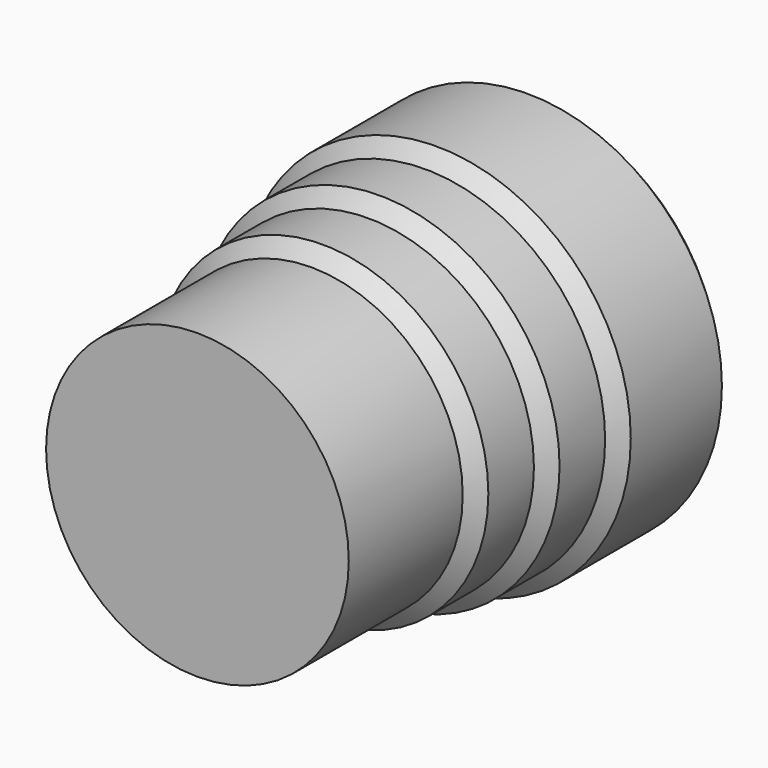
from build123d import *

# Parameters (mm, degrees)
F0_R     = 69.2237369755
F1_DEPTH = 50.8
F2_SIZE  = 5.08
F3_DEPTH = 25.4
F4_SIZE  = 5.08
F5_DEPTH = 25.4
F6_SIZE  = 5.08
F7_DEPTH = 50.8


with BuildPart() as f1:
    # F0 (on Front) → F1 (new body)
    with BuildSketch(Plane.XZ):
        with Locations((-16.0285290331, 36.5865901113)):
            Circle(F0_R)
    extrude(amount=F1_DEPTH)

    # F2
    f2_edges = [f1.edges().sort_by_distance(p)[0] for p in [
        (53.195208, -25.4, 36.58659),
        (-85.252266, 0, 36.58659),
        (-85.252266, -50.8, 36.58659),
    ]]
    chamfer(f2_edges, length=F2_SIZE)

    # F3 (add): a face of the model
    f3_faces = [f1.faces().sort_by_distance(p)[0] for p in [
        (-16.0285290331, -50.8, 36.5865901113),
    ]]
    extrude(f3_faces, amount=F3_DEPTH)

    # F4
    f4_edges = [f1.edges().sort_by_distance(p)[0] for p in [
        (-80.172266, -76.2, 36.58659),
    ]]
    chamfer(f4_edges, length=F4_SIZE)

    # F5 (add): a face of the model
    f5_faces = [f1.faces().sort_by_distance(p)[0] for p in [
        (-16.0285290331, -76.2, 36.5865901113),
    ]]
    extrude(f5_faces, amount=F5_DEPTH)

    # F6
    f6_edges = [f1.edges().sort_by_distance(p)[0] for p in [
        (-75.092266, -101.6, 36.58659),
    ]]
    chamfer(f6_edges, length=F6_SIZE)

    # F7 (add): a face of the model
    f7_faces = [f1.faces().sort_by_distance(p)[0] for p in [
        (-16.0285290331, -101.6, 36.5865901113),
    ]]
    extrude(f7_faces, amount=F7_DEPTH)


solid = f1.part
